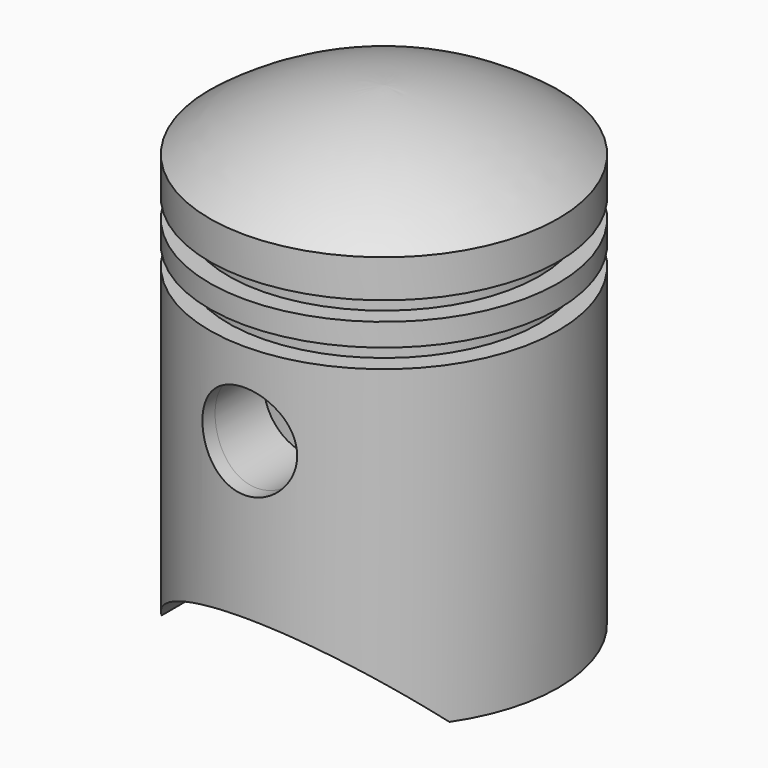
from build123d import *

# Parameters (mm, degrees)
F3_DEPTH = 32.5
F4_R     = 6.25
F5_DEPTH = 30
F7_R     = 7.25
F7_R_2   = 6.25


# Not quite as in the source:
# - a pattern or mirror of a feature is missing from the dataset's text; its kind, count and spacing are read off the source's solid


with BuildPart() as f1:
    # F0 (on Front) → F1 (revolve)
    with BuildSketch(Plane.XZ):
        with BuildLine():
            ThreePointArc((23, 54.5), (12.1235156232, 60.2923848686), (0, 62.4991933782))
            Line((0, 62.4991933782), (0, 60.498556228))
            ThreePointArc((0, 60.498556228), (10.0731822074, 59.3307401104), (19.4210526316, 55.4000769604))
            Line((19.4210526316, 55.4000769604), (19.4210526316, 39.8824422241))
            Line((19.4210526316, 39.8824422241), (19.4210526316, 39.7824422264))
            Line((19.4210526316, 39.7824422264), (21, 39.7824422264))
            Line((21, 39.7824422264), (21, 0))
            Line((21, 0), (23, 0))
            Line((23, 0), (23, 41.5))
            Line((23, 41.5), (20.5, 41.5))
            Line((20.5, 41.5), (20.5, 44))
            Line((20.5, 44), (23, 44))
            Line((23, 44), (23, 47))
            Line((23, 47), (20.5, 47))
            Line((20.5, 47), (20.5, 49.5))
            Line((20.5, 49.5), (23, 49.5))
            Line((23, 49.5), (23, 54.5))
        make_face()
    revolve(axis=Axis((0, 0, 61.4988748031), (0, 0, -1)))

    # F2 (on Front) → F3 (cut, symmetric)
    with BuildSketch(Plane.XZ):
        with BuildLine():
            ThreePointArc((19, 0), (0, 10), (-19, 0))
            Line((-19, 0), (19, 0))
        make_face()
    extrude(amount=F3_DEPTH, both=True, mode=Mode.SUBTRACT)

    # F4 (on Front) → F5 (cut, symmetric)
    with BuildSketch(Plane.XZ):
        with Locations((0, 30.4991933782)):
            Circle(F4_R)
    extrude(amount=F5_DEPTH, both=True, mode=Mode.SUBTRACT)

    # F7 (on offset) → F8 (join, up to the next surface of F1)
    with BuildSketch(Plane.XZ.offset(12)):
        with Locations((0, 30.4991933782)):
            Circle(F7_R)
        with Locations((0, 30.4991933782)):
            Circle(F7_R_2, mode=Mode.SUBTRACT)
    f8 = extrude(until=Until.NEXT)

    # F8_copies: F8 across plane
    add(f8.mirror(Plane.ZX))


solid = f1.part
